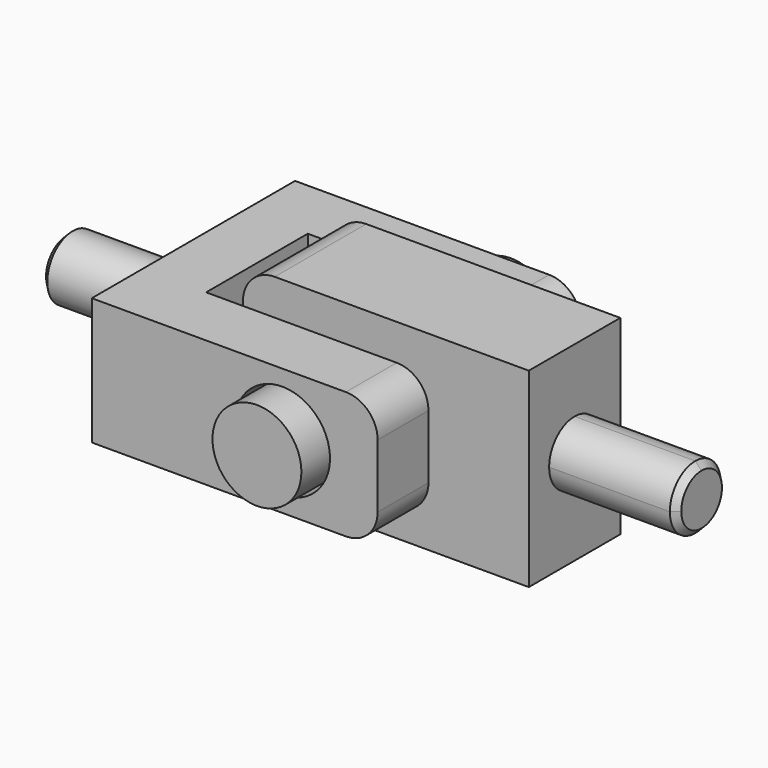
from build123d import *

# Parameters (mm, degrees)
F0_R          = 5
F1_DEPTH      = 20
F3_DEPTH      = 20
F4_R          = 5
F6_D          = 15
F7_SIZE       = 1
F5_R          = 7
F8_DEPTH      = 45
F8_DEPTH_BACK = 5
F9_START      = 11
F5_R_2        = 7.5
F9_DEPTH      = 18
F10_R         = 5
F11_START     = 15
F5_W          = 20
F5_H          = 10
F11_DEPTH     = 10
F12_R         = 4.99999
F13_SIZE      = 1


# Not quite as in the source:
# - a fillet or chamfer is up to 0.001 mm smaller than in the source, because OpenCascade refuses the exact size
# - a feature names something its author has since deleted; it is built from what else it names


with BuildPart() as f1:
    # F0 (on Right) → F1 (new body)
    with BuildSketch(Plane.YZ):
        with Locations((-20, -10)):
            Circle(F0_R)
    extrude(amount=-F1_DEPTH)

    # F2 (on Top) → F3 (join)
    with BuildSketch(Plane.XY):
        Polygon((45, 0), (0, 0), (0, -40), (45, -40), (45, -30), (15, -30), (10, -30), (10, -10), (15, -10), (45, -10), align=None)
    extrude(amount=-F3_DEPTH)

    # F4
    f4_edges = [f1.edges().sort_by_distance(p)[0] for p in [
        (45, -35, 0),
        (45, -5, 0),
        (45, -35, -20),
        (45, -5, -20),
    ]]
    fillet(f4_edges, radius=F4_R)

    # F6 (through all)
    with Locations(Plane(origin=(0, 0, 0), x_dir=(1, 0, 0), z_dir=(0, 1, 0))):
        with Locations((30, 10)):
            Hole(F6_D / 2)

    # F7
    f7_edges = [f1.edges().sort_by_distance(p)[0] for p in [
        (-20, -25, -10),
    ]]
    chamfer(f7_edges, length=F7_SIZE)


with BuildPart() as f8:
    # F5 (on Front) → F8 (new body, two sides)
    with BuildSketch(Plane.XZ) as f8_sk:
        with Locations((30, -10)):
            Circle(F5_R)
    extrude(amount=F8_DEPTH)
    extrude(f8_sk.sketch, amount=-F8_DEPTH_BACK)


with BuildPart() as f9:
    # F5 (on Front) → F9 (new body)
    with BuildSketch(Plane.XZ.offset(F9_START)):
        Polygon((60, 5), (15, 5), (15, -25), (60, -25), (60, -15), (60, -5), align=None)
        with Locations((30, -10)):
            Circle(F5_R_2, mode=Mode.SUBTRACT)
    extrude(amount=F9_DEPTH)

    # F10
    f10_edges = [f9.edges().sort_by_distance(p)[0] for p in [
        (15, -20, 5),
        (15, -20, -25),
    ]]
    fillet(f10_edges, radius=F10_R)

    # F5 (on Front) → F11 (join)
    with BuildSketch(Plane.XZ.offset(F11_START)):
        with Locations((70, -10)):
            Rectangle(F5_W, F5_H)
    extrude(amount=F11_DEPTH)

    # F12 (radius 5 in the source; OpenCascade refuses exactly that, so slightly less here)
    f12_edges = [f9.edges().sort_by_distance(p)[0] for p in [
        (70, -25, -5),
        (70, -15, -5),
        (70, -15, -15),
        (70, -25, -15),
    ]]
    fillet(f12_edges, radius=F12_R)

    # F13
    f13_edges = [f9.edges().sort_by_distance(p)[0] for p in [
        (80, -20, -15),
        (80, -16.464463, -13.535537),
        (80, -23.535537, -13.535537),
        (80, -15, -10),
        (80, -25, -10),
        (80, -16.464463, -6.464463),
        (80, -23.535537, -6.464463),
        (80, -20, -5),
    ]]
    chamfer(f13_edges, length=F13_SIZE)


solid = Compound([f1.part, f8.part, f9.part])
